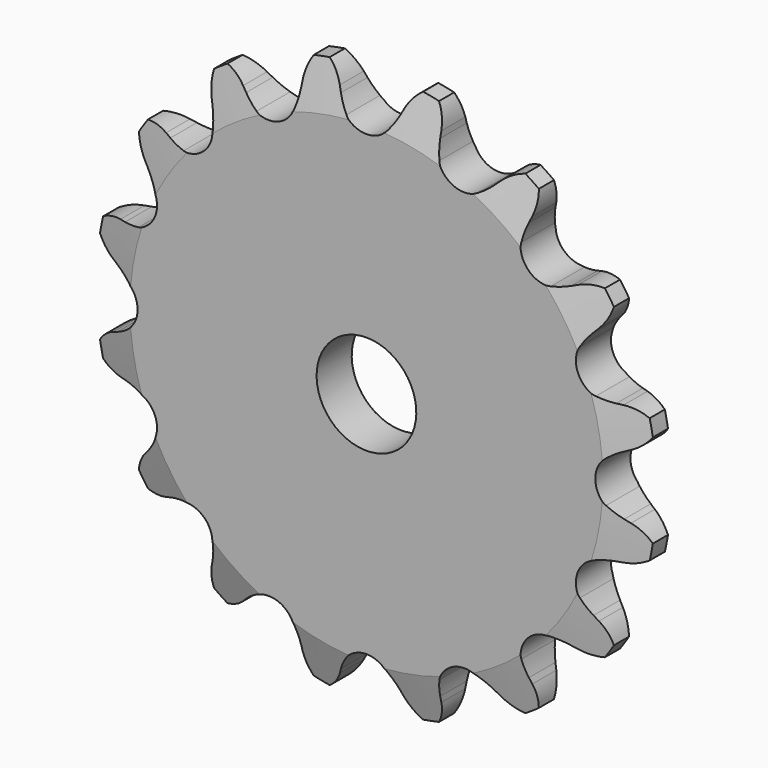
from build123d import *

# Parameters (mm, degrees)
F0_W     = 2.794
F0_H     = 9.525
F0_H_2   = 5.1562
F2_SIZE2 = 2.794
F2_SIZE  = 0.79375
F4_DEPTH = 2.795


with BuildPart() as f1:
    # F0 (on Right) → F1 (revolve)
    with BuildSketch(Plane.YZ):
        with Locations((1.397, 7.9375)):
            Rectangle(F0_W, F0_H)
        with Locations((1.397, 15.2781)):
            Rectangle(F0_W, F0_H_2)
    revolve(axis=Axis((0, 5.8612824179, 0), (0, 1, 0)))

    # F2
    f2_edges = [f1.edges().sort_by_distance(p)[0] for p in [
        (0, 0, -17.8562),
        (0, 2.794, -17.8562),
    ]]
    f2_side = f1.faces().sort_by_distance((0, 1.397, -17.8562))[0]
    chamfer(f2_edges, length=F2_SIZE, length2=F2_SIZE2, reference=f2_side)

    # F3 (on face) → F4 (intersect, through all)
    with BuildSketch(Plane.XZ):
        with BuildLine():
            ThreePointArc((-1.3242360534, 15.2122382035), (-1.6399658803, 15.6610598977), (-1.8965305961, 16.1461380185))
            Line((-1.8965305961, 16.1461380185), (-2.0521895801, 16.4916881494))
            ThreePointArc((-2.0521895801, 16.4916881494), (-2.6667426734, 17.3543615176), (-3.5639671459, 17.9172727811))
            ThreePointArc((-3.5639671459, 17.9172727811), (-4.1774776577, 17.0538576454), (-4.4151198766, 16.0216720902))
            Line((-4.4151198766, 16.0216720902), (-4.4266937158, 15.6428572825))
            ThreePointArc((-4.4266937158, 15.6428572825), (-4.4780972453, 15.0965204689), (-4.5980369437, 14.5610387181))
            ThreePointArc((-4.5980369437, 14.5610387181), (-5.5783993546, 13.4674473782), (-7.0449061157, 13.5475123217))
            ThreePointArc((-7.0449061157, 13.5475123217), (-7.5083590669, 13.8413449249), (-7.9310253169, 14.1913156063))
            Line((-7.9310253169, 14.1913156063), (-8.2070717764, 14.4509941854))
            ThreePointArc((-8.2070717764, 14.4509941854), (-9.1049756064, 15.0128211664), (-10.1493197471, 15.1895304207))
            ThreePointArc((-10.1493197471, 15.1895304207), (-10.3857148843, 14.1570585403), (-10.2102673553, 13.112501692))
            Line((-10.2102673553, 13.112501692), (-10.0759940376, 12.7580933281))
            ThreePointArc((-10.0759940376, 12.7580933281), (-9.9144106593, 12.2336726491), (-9.8203004974, 11.693053084))
            ThreePointArc((-9.8203004974, 11.693053084), (-10.3075379758, 10.3075379758), (-11.693053084, 9.8203004974))
            ThreePointArc((-11.693053084, 9.8203004974), (-12.2336726491, 9.9144106593), (-12.7580933281, 10.0759940376))
            Line((-12.7580933281, 10.0759940376), (-13.112501692, 10.2102673553))
            ThreePointArc((-13.112501692, 10.2102673553), (-14.1570585403, 10.3857148843), (-15.1895304207, 10.1493197471))
            ThreePointArc((-15.1895304207, 10.1493197471), (-15.0128211664, 9.1049756064), (-14.4509941854, 8.2070717764))
            Line((-14.4509941854, 8.2070717764), (-14.1913156063, 7.9310253169))
            ThreePointArc((-14.1913156063, 7.9310253169), (-13.8413449249, 7.5083590669), (-13.5475123217, 7.0449061157))
            ThreePointArc((-13.5475123217, 7.0449061157), (-13.4674473782, 5.5783993546), (-14.5610387181, 4.5980369437))
            ThreePointArc((-14.5610387181, 4.5980369437), (-15.0965204689, 4.4780972453), (-15.6428572825, 4.4266937158))
            Line((-15.6428572825, 4.4266937158), (-16.0216720902, 4.4151198766))
            ThreePointArc((-16.0216720902, 4.4151198766), (-17.0538576454, 4.1774776577), (-17.9172727811, 3.5639671459))
            ThreePointArc((-17.9172727811, 3.5639671459), (-17.3543615176, 2.6667426734), (-16.4916881494, 2.0521895801))
            Line((-16.4916881494, 2.0521895801), (-16.1461380185, 1.8965305961))
            ThreePointArc((-16.1461380185, 1.8965305961), (-15.6610598977, 1.6399658803), (-15.2122382035, 1.3242360534))
            ThreePointArc((-15.2122382035, 1.3242360534), (-14.57706, 0), (-15.2122382035, -1.3242360534))
            ThreePointArc((-15.2122382035, -1.3242360534), (-15.6610598977, -1.6399658803), (-16.1461380185, -1.8965305961))
            Line((-16.1461380185, -1.8965305961), (-16.4916881494, -2.0521895801))
            ThreePointArc((-16.4916881494, -2.0521895801), (-17.3543615176, -2.6667426734), (-17.9172727811, -3.5639671459))
            ThreePointArc((-17.9172727811, -3.5639671459), (-17.0538576454, -4.1774776577), (-16.0216720902, -4.4151198766))
            Line((-16.0216720902, -4.4151198766), (-15.6428572825, -4.4266937158))
            ThreePointArc((-15.6428572825, -4.4266937158), (-15.0965204689, -4.4780972453), (-14.5610387181, -4.5980369437))
            ThreePointArc((-14.5610387181, -4.5980369437), (-13.4674473782, -5.5783993546), (-13.5475123217, -7.0449061157))
            ThreePointArc((-13.5475123217, -7.0449061157), (-13.8413449249, -7.5083590669), (-14.1913156063, -7.9310253169))
            Line((-14.1913156063, -7.9310253169), (-14.4509941854, -8.2070717764))
            ThreePointArc((-14.4509941854, -8.2070717764), (-15.0128211664, -9.1049756064), (-15.1895304207, -10.1493197471))
            ThreePointArc((-15.1895304207, -10.1493197471), (-14.1570585403, -10.3857148843), (-13.112501692, -10.2102673553))
            Line((-13.112501692, -10.2102673553), (-12.7580933281, -10.0759940376))
            ThreePointArc((-12.7580933281, -10.0759940376), (-12.2336726491, -9.9144106593), (-11.693053084, -9.8203004974))
            ThreePointArc((-11.693053084, -9.8203004974), (-10.3075379758, -10.3075379758), (-9.8203004974, -11.693053084))
            ThreePointArc((-9.8203004974, -11.693053084), (-9.9144106593, -12.2336726491), (-10.0759940376, -12.7580933281))
            Line((-10.0759940376, -12.7580933281), (-10.2102673553, -13.112501692))
            ThreePointArc((-10.2102673553, -13.112501692), (-10.3857148843, -14.1570585403), (-10.1493197471, -15.1895304207))
            ThreePointArc((-10.1493197471, -15.1895304207), (-9.1049756064, -15.0128211664), (-8.2070717764, -14.4509941854))
            Line((-8.2070717764, -14.4509941854), (-7.9310253169, -14.1913156063))
            ThreePointArc((-7.9310253169, -14.1913156063), (-7.5083590669, -13.8413449249), (-7.0449061157, -13.5475123217))
            ThreePointArc((-7.0449061157, -13.5475123217), (-5.5783993546, -13.4674473782), (-4.5980369437, -14.5610387181))
            ThreePointArc((-4.5980369437, -14.5610387181), (-4.4780972453, -15.0965204689), (-4.4266937158, -15.6428572825))
            Line((-4.4266937158, -15.6428572825), (-4.4151198766, -16.0216720902))
            ThreePointArc((-4.4151198766, -16.0216720902), (-4.1774776577, -17.0538576454), (-3.5639671459, -17.9172727811))
            ThreePointArc((-3.5639671459, -17.9172727811), (-2.6667426734, -17.3543615176), (-2.0521895801, -16.4916881494))
            Line((-2.0521895801, -16.4916881494), (-1.8965305961, -16.1461380185))
            ThreePointArc((-1.8965305961, -16.1461380185), (-1.6399658803, -15.6610598977), (-1.3242360534, -15.2122382035))
            ThreePointArc((-1.3242360534, -15.2122382035), (0, -14.57706), (1.3242360534, -15.2122382035))
            ThreePointArc((1.3242360534, -15.2122382035), (1.6399658803, -15.6610598977), (1.8965305961, -16.1461380185))
            Line((1.8965305961, -16.1461380185), (2.0521895801, -16.4916881494))
            ThreePointArc((2.0521895801, -16.4916881494), (2.6667426734, -17.3543615176), (3.5639671459, -17.9172727811))
            ThreePointArc((3.5639671459, -17.9172727811), (4.1774776577, -17.0538576454), (4.4151198766, -16.0216720902))
            Line((4.4151198766, -16.0216720902), (4.4266937158, -15.6428572825))
            ThreePointArc((4.4266937158, -15.6428572825), (4.4780972453, -15.0965204689), (4.5980369437, -14.5610387181))
            ThreePointArc((4.5980369437, -14.5610387181), (5.5783993546, -13.4674473782), (7.0449061157, -13.5475123217))
            ThreePointArc((7.0449061157, -13.5475123217), (7.5083590669, -13.8413449249), (7.9310253169, -14.1913156063))
            Line((7.9310253169, -14.1913156063), (8.2070717764, -14.4509941854))
            ThreePointArc((8.2070717764, -14.4509941854), (9.1049756064, -15.0128211664), (10.1493197471, -15.1895304207))
            ThreePointArc((10.1493197471, -15.1895304207), (10.3857148843, -14.1570585403), (10.2102673553, -13.112501692))
            Line((10.2102673553, -13.112501692), (10.0759940376, -12.7580933281))
            ThreePointArc((10.0759940376, -12.7580933281), (9.9144106593, -12.2336726491), (9.8203004974, -11.693053084))
            ThreePointArc((9.8203004974, -11.693053084), (10.3075379758, -10.3075379758), (11.693053084, -9.8203004974))
            ThreePointArc((11.693053084, -9.8203004974), (12.2336726491, -9.9144106593), (12.7580933281, -10.0759940376))
            Line((12.7580933281, -10.0759940376), (13.112501692, -10.2102673553))
            ThreePointArc((13.112501692, -10.2102673553), (14.1570585403, -10.3857148843), (15.1895304207, -10.1493197471))
            ThreePointArc((15.1895304207, -10.1493197471), (15.0128211664, -9.1049756064), (14.4509941854, -8.2070717764))
            Line((14.4509941854, -8.2070717764), (14.1913156063, -7.9310253169))
            ThreePointArc((14.1913156063, -7.9310253169), (13.8413449249, -7.5083590669), (13.5475123217, -7.0449061157))
            ThreePointArc((13.5475123217, -7.0449061157), (13.4674473782, -5.5783993546), (14.5610387181, -4.5980369437))
            ThreePointArc((14.5610387181, -4.5980369437), (15.0965204689, -4.4780972453), (15.6428572825, -4.4266937158))
            Line((15.6428572825, -4.4266937158), (16.0216720902, -4.4151198766))
            ThreePointArc((16.0216720902, -4.4151198766), (17.0538576454, -4.1774776577), (17.9172727811, -3.5639671459))
            ThreePointArc((17.9172727811, -3.5639671459), (17.3543615176, -2.6667426734), (16.4916881494, -2.0521895801))
            Line((16.4916881494, -2.0521895801), (16.1461380185, -1.8965305961))
            ThreePointArc((16.1461380185, -1.8965305961), (15.6610598977, -1.6399658803), (15.2122382035, -1.3242360534))
            ThreePointArc((15.2122382035, -1.3242360534), (14.57706, 0), (15.2122382035, 1.3242360534))
            ThreePointArc((15.2122382035, 1.3242360534), (15.6610598977, 1.6399658803), (16.1461380185, 1.8965305961))
            Line((16.1461380185, 1.8965305961), (16.4916881494, 2.0521895801))
            ThreePointArc((16.4916881494, 2.0521895801), (17.3543615176, 2.6667426734), (17.9172727811, 3.5639671459))
            ThreePointArc((17.9172727811, 3.5639671459), (17.0538576454, 4.1774776577), (16.0216720902, 4.4151198766))
            Line((16.0216720902, 4.4151198766), (15.6428572825, 4.4266937158))
            ThreePointArc((15.6428572825, 4.4266937158), (15.0965204689, 4.4780972453), (14.5610387181, 4.5980369437))
            ThreePointArc((14.5610387181, 4.5980369437), (13.4674473782, 5.5783993546), (13.5475123217, 7.0449061157))
            ThreePointArc((13.5475123217, 7.0449061157), (13.8413449249, 7.5083590669), (14.1913156063, 7.9310253169))
            Line((14.1913156063, 7.9310253169), (14.4509941854, 8.2070717764))
            ThreePointArc((14.4509941854, 8.2070717764), (15.0128211664, 9.1049756064), (15.1895304207, 10.1493197471))
            ThreePointArc((15.1895304207, 10.1493197471), (14.1570585403, 10.3857148843), (13.112501692, 10.2102673553))
            Line((13.112501692, 10.2102673553), (12.7580933281, 10.0759940376))
            ThreePointArc((12.7580933281, 10.0759940376), (12.2336726491, 9.9144106593), (11.693053084, 9.8203004974))
            ThreePointArc((11.693053084, 9.8203004974), (10.3075379758, 10.3075379758), (9.8203004974, 11.693053084))
            ThreePointArc((9.8203004974, 11.693053084), (9.9144106593, 12.2336726491), (10.0759940376, 12.7580933281))
            Line((10.0759940376, 12.7580933281), (10.2102673553, 13.112501692))
            ThreePointArc((10.2102673553, 13.112501692), (10.3857148843, 14.1570585403), (10.1493197471, 15.1895304207))
            ThreePointArc((10.1493197471, 15.1895304207), (9.1049756064, 15.0128211664), (8.2070717764, 14.4509941854))
            Line((8.2070717764, 14.4509941854), (7.9310253169, 14.1913156063))
            ThreePointArc((7.9310253169, 14.1913156063), (7.5083590669, 13.8413449249), (7.0449061157, 13.5475123217))
            ThreePointArc((7.0449061157, 13.5475123217), (5.5783993546, 13.4674473782), (4.5980369437, 14.5610387181))
            ThreePointArc((4.5980369437, 14.5610387181), (4.4780972453, 15.0965204689), (4.4266937158, 15.6428572825))
            Line((4.4266937158, 15.6428572825), (4.4151198766, 16.0216720902))
            ThreePointArc((4.4151198766, 16.0216720902), (4.1774776577, 17.0538576454), (3.5639671459, 17.9172727811))
            ThreePointArc((3.5639671459, 17.9172727811), (2.6667426734, 17.3543615176), (2.0521895801, 16.4916881494))
            Line((2.0521895801, 16.4916881494), (1.8965305961, 16.1461380185))
            ThreePointArc((1.8965305961, 16.1461380185), (1.6399658803, 15.6610598977), (1.3242360534, 15.2122382035))
            ThreePointArc((1.3242360534, 15.2122382035), (0, 14.57706), (-1.3242360534, 15.2122382035))
        make_face()
    extrude(amount=-F4_DEPTH, mode=Mode.INTERSECT)


solid = f1.part
